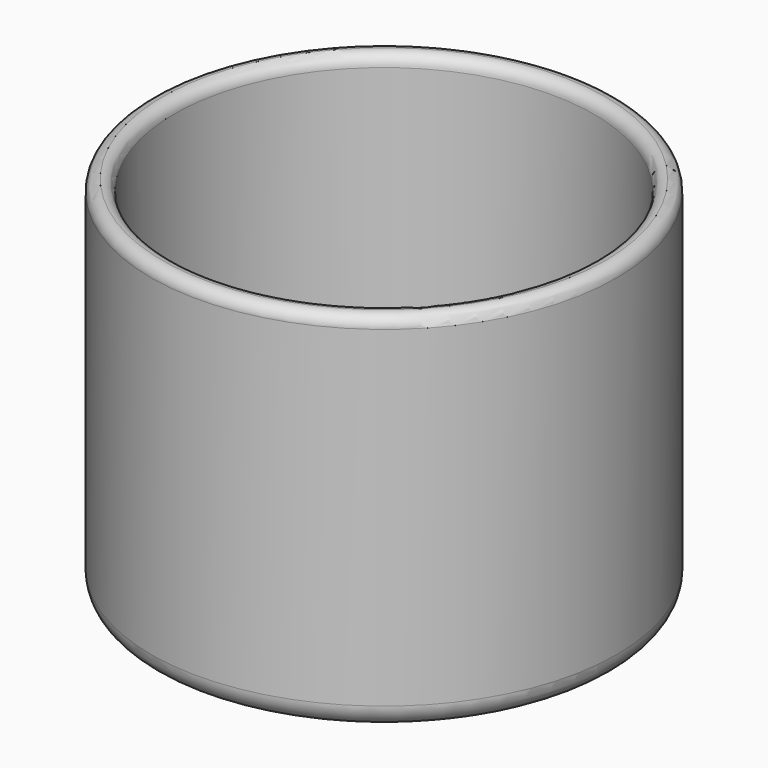
from build123d import *

# Parameters (mm, degrees)
F0_R      = 51.7494214311
F1_DEPTH  = 76.2
F2_T      = -5.08
F1_FACE_R = 51.7494214311
F3_DEPTH  = 5.08
F4_R      = 2.53999
F5_R      = 5.08
F6_R      = 5.07999


# Not quite as in the source:
# - a fillet or chamfer is up to 0.001 mm smaller than in the source, because OpenCascade refuses the exact size


with BuildPart() as f1:
    # F0 (on Top) → F1 (new body)
    with BuildSketch(Plane.XY):
        Circle(F0_R)
    extrude(amount=F1_DEPTH)

    # F2
    f2_openings = [f1.faces().sort_by_distance(p)[0] for p in [
        (0, 0, 76.2),
    ]]
    offset(amount=F2_T, openings=f2_openings)

    # F0 (on Top) + F1_face (on face) → F3 (join)
    with BuildSketch(Plane.XY):
        Circle(F0_R)
    with BuildSketch(Plane(origin=(0, 0, 0), x_dir=(1, 0, 0), z_dir=(0, 0, -1))):
        Circle(F1_FACE_R)
    extrude(amount=-F3_DEPTH, dir=(0, 0, 1))

    # F4 (radius 2.54 in the source; OpenCascade refuses exactly that, so slightly less here)
    f4_edges = [f1.edges().sort_by_distance(p)[0] for p in [
        (-51.749421, 0, 76.2),
        (-46.669421, 0, 76.2),
    ]]
    fillet(f4_edges, radius=F4_R)

    # F5
    f5_edges = [f1.edges().sort_by_distance(p)[0] for p in [
        (-46.669421, 0, 5.08),
    ]]
    fillet(f5_edges, radius=F5_R)

    # F6 (radius 5.08 in the source; OpenCascade refuses exactly that, so slightly less here)
    f6_edges = [f1.edges().sort_by_distance(p)[0] for p in [
        (-51.749421, 0, -5.08),
    ]]
    fillet(f6_edges, radius=F6_R)


solid = f1.part
